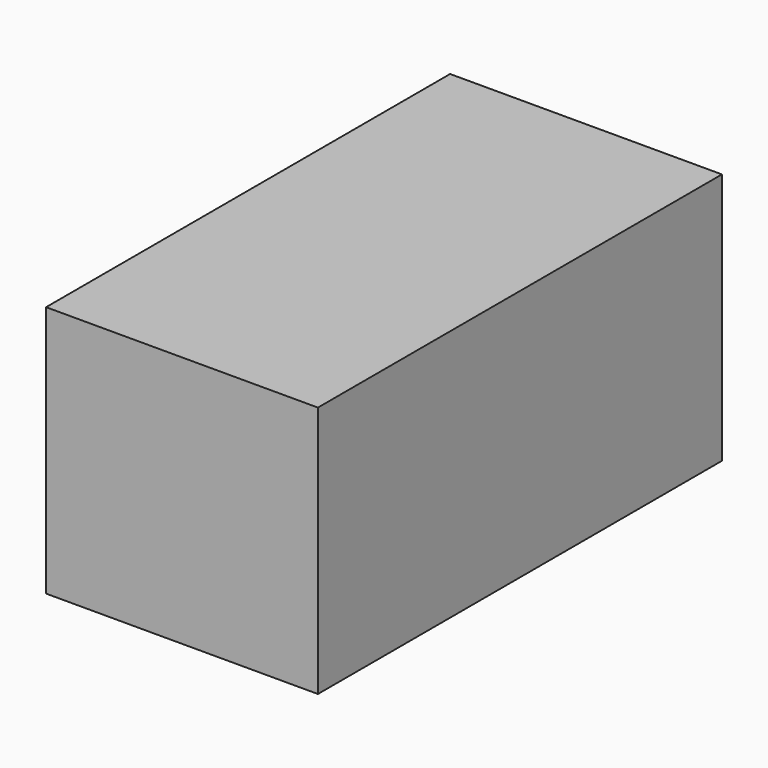
from build123d import *

# Parameters (mm, degrees)
F0_W     = 13.6721115559
F0_H     = 12.6828635111
F1_DEPTH = 25.4


with BuildPart() as f1:
    # F0 (on Front) → F1 (new body)
    with BuildSketch(Plane.XZ):
        with Locations((-6.836055778, 6.3414317556)):
            Rectangle(F0_W, F0_H)
    extrude(amount=F1_DEPTH)


solid = f1.part
